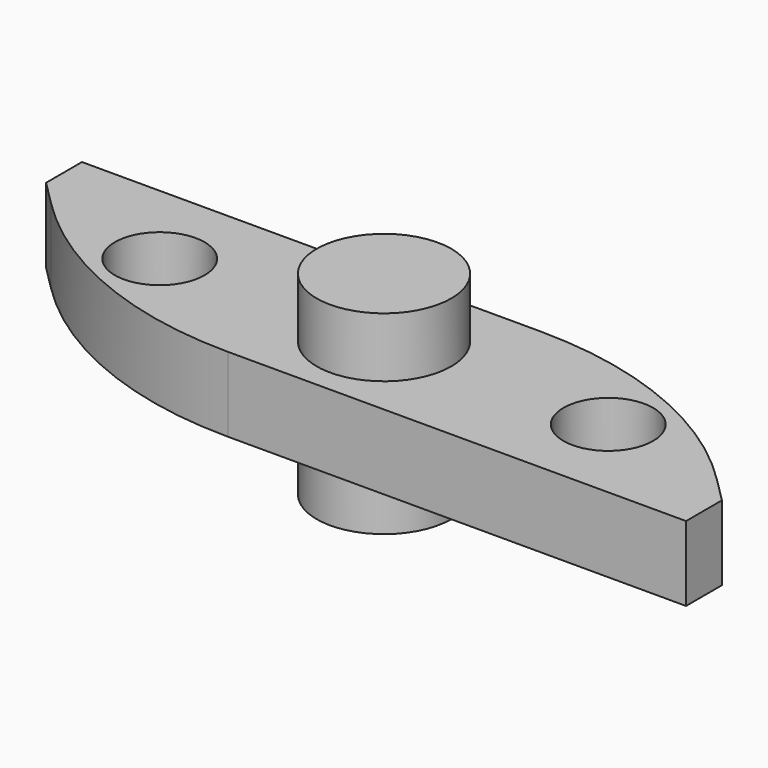
from build123d import *

# Parameters (mm, degrees)
F0_W          = 500
F0_H          = 120
F0_R          = 30
F1_DEPTH      = 25
F2_R          = 45
F3_DEPTH      = 40
F3_DEPTH_BACK = 90
F4_SIZE       = 90
F5_R          = 250


with BuildPart() as f1:
    # F0 (on Top) → F1 (new body, symmetric)
    with BuildSketch(Plane.XY):
        Rectangle(F0_W, F0_H)
        with Locations((-150, 0)):
            Circle(F0_R, mode=Mode.SUBTRACT)
        with Locations((150, 0)):
            Circle(F0_R, mode=Mode.SUBTRACT)
    extrude(amount=F1_DEPTH, both=True)

    # F2 (on face) → F3 (join, two sides)
    with BuildSketch(Plane.XY.offset(25)) as f3_sk:
        Circle(F2_R)
    extrude(amount=F3_DEPTH)
    extrude(f3_sk.sketch, amount=-F3_DEPTH_BACK)

    # F4
    f4_edges = [f1.edges().sort_by_distance(p)[0] for p in [
        (-250, -60, 0),
        (250, 60, 0),
    ]]
    chamfer(f4_edges, length=F4_SIZE)

    # F5
    f5_edges = [f1.edges().sort_by_distance(p)[0] for p in [
        (-160, -60, 0),
        (160, 60, 0),
    ]]
    fillet(f5_edges, radius=F5_R)


solid = f1.part
